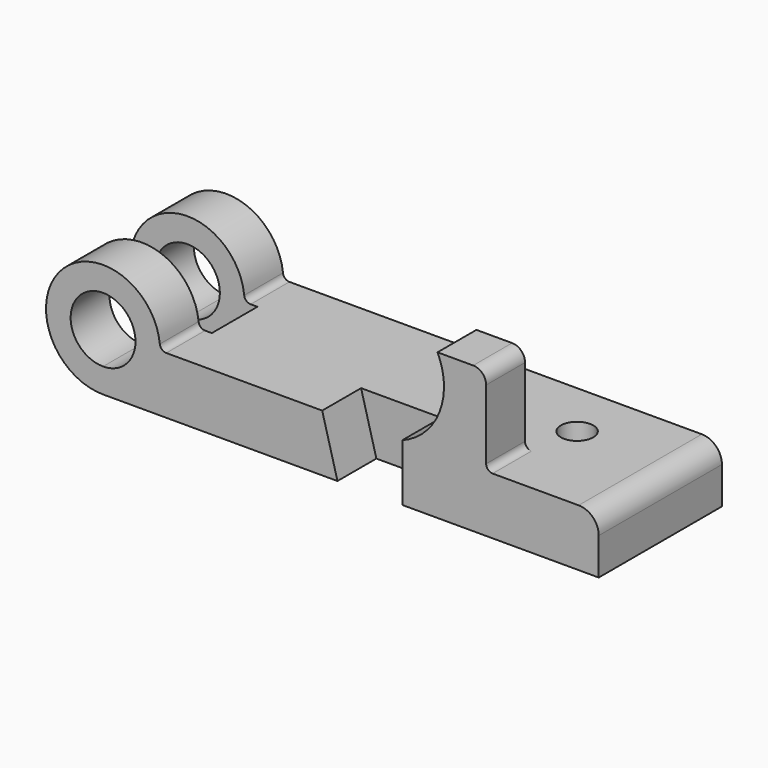
from build123d import *

# Parameters (mm, degrees)
F1_DEPTH = 30.1625
F3_DEPTH = 19.05
F4_DEPTH = 19.05
F5_R     = 5.08
F6_R     = 2.54
F8_R     = 7.874
F7_W     = 54.254862
F7_H     = 22.3266
F7_R     = 6.35
F9_DEPTH = 47.752


with BuildPart() as f1:
    # F0 (on Front) → F1 (new body, symmetric)
    with BuildSketch(Plane.XZ):
        with BuildLine():
            ThreePointArc((0, -12.7), (-8.980256, 8.980256), (12.7, 0))
            Line((12.7, 0), (22.352, 0))
            ThreePointArc((22.352, 0), (-15.805251, 15.805251), (0, -22.352))
            Line((0, -22.352), (0, -12.7))
        make_face()
        with BuildLine():
            Line((22.352, 0), (12.7, 0))
            ThreePointArc((12.7, 0), (8.980256, -8.980256), (0, -12.7))
            Line((0, -12.7), (0, -22.352))
            Line((0, -22.352), (91.8464, -22.352))
            Line((91.8464, -22.352), (85.852, 0))
            Line((85.852, 0), (22.352, 0))
        make_face()
        Polygon((117.2464, 0), (85.852, 0), (91.8464, -22.352), (117.2464, -22.352), align=None)
        Polygon((150.0886, 0), (117.2464, 0), (117.2464, -22.352), (194.2084, -22.352), (194.2084, 0), align=None)
    extrude(amount=F1_DEPTH, both=True)

    # F2 (on face) → F3 (cut)
    with BuildSketch(Plane.XZ.offset(30.1625)):
        Polygon((117.2464, -22.352), (117.2464, 0), (85.852, 0), (91.8464, -22.352), align=None)
    extrude(amount=-F3_DEPTH, mode=Mode.SUBTRACT)

    # F2 (on face) → F4 (join)
    with BuildSketch(Plane.XZ.offset(30.1625)):
        with BuildLine():
            Line((150.0886, 34.798), (131.0386, 34.798))
            ThreePointArc((131.0386, 34.798), (131.791567, 14.367289), (117.2464, 0))
            Line((117.2464, 0), (150.0886, 0))
            Line((150.0886, 0), (150.0886, 34.798))
        make_face()
    extrude(amount=-F4_DEPTH)

    # F5
    f5_edges = [f1.edges().sort_by_distance(p)[0] for p in [
        (150.0886, -20.6375, 34.798),
    ]]
    fillet(f5_edges, radius=F5_R)

    # F6
    f6_edges = [f1.edges().sort_by_distance(p)[0] for p in [
        (150.0886, -20.6375, 0),
        (22.352, 0, 0),
    ]]
    fillet(f6_edges, radius=F6_R)

    # F8
    f8_edges = [f1.edges().sort_by_distance(p)[0] for p in [
        (194.2084, 0, 0),
    ]]
    fillet(f8_edges, radius=F8_R)

    # F7 (on Top) → F9 (cut, symmetric)
    with BuildSketch(Plane.XY):
        with Locations((0.283614, 0)):
            Rectangle(F7_W, F7_H)
        with Locations((155.3464, 7.8105)):
            Circle(F7_R)
    extrude(amount=F9_DEPTH, both=True, mode=Mode.SUBTRACT)


solid = f1.part
